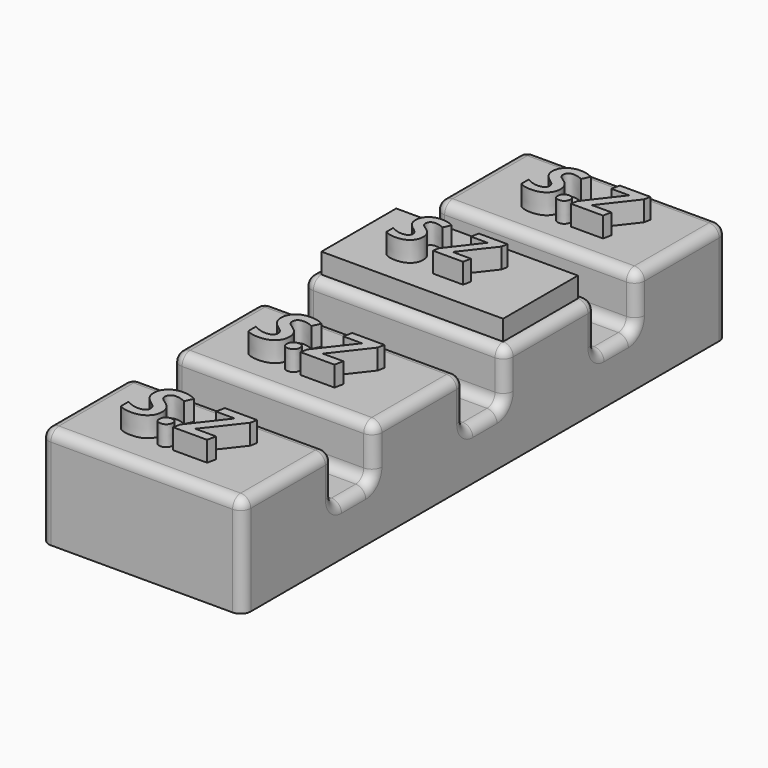
from build123d import *

# Parameters (mm, degrees)
F0_W           = 25.4
F0_H           = 76.2
F1_DEPTH       = 12.7
F2_W           = 6.35
F2_H           = 12.7
F3_DEPTH       = 25.401
F4_F1_R        = 1.27
F4_F2_R        = 1.27
F5_T           = -2.54
F6_TEXT_SIZE   = 7.9179738855
F6_TEXT_SIZE_2 = 8.9047935843
F6_TEXT_SIZE_3 = 8.906235194
F7_DEPTH       = 2.54
F8_TEXT_SIZE   = 8.433056064
F3_FACE_W      = 22.86
F3_FACE_H      = 11.7602
F9_DEPTH       = 2.54


# Not quite as in the source:
# - Text() gives the source's letters only with a copy of the font that has no kerning and outlines rounded to 1/6400 em; it was checked with that copy


with BuildPart() as f1:
    # F0 (on Top) → F1 (new body)
    with BuildSketch(Plane.XY):
        Rectangle(F0_W, F0_H)
    extrude(amount=F1_DEPTH)

    # F2 (on face) → F3 (cut, through all)
    with BuildSketch(Plane.YZ.offset(12.7)):
        with Locations((0, 12.7)):
            Rectangle(F2_W, F2_H)
        with Locations((-20.6502, 12.7)):
            Rectangle(F2_W, F2_H)
        with Locations((20.6502, 12.7)):
            Rectangle(F2_W, F2_H)
    extrude(amount=-F3_DEPTH, mode=Mode.SUBTRACT)

    # F4: fillet of radius 1.27 on 32 edges, made by hand

    # F4_f1
    f4_f1_edges = [f1.edges().sort_by_distance(p)[0] for p in [
        (0, -23.8252, 6.35),
        (0, 3.175, 6.35),
        (0, -3.175, 6.35),
        (0, 23.8252, 6.35),
        (0, 17.4752, 6.35),
        (0, -17.4752, 6.35),
    ]]
    fillet(f4_f1_edges, radius=F4_F1_R)

    # F4_f2
    f4_f2_edges = [f1.edges().sort_by_distance(p)[0] for p in [
        (12.7, -30.9626, 12.7),
        (0, -38.1, 12.7),
        (-12.7, -30.9626, 12.7),
        (0, -23.8252, 12.7),
        (12.7, -10.3251, 12.7),
        (0, -17.4752, 12.7),
        (-12.7, -10.3251, 12.7),
        (0, -3.175, 12.7),
        (12.7, 10.3251, 12.7),
        (0, 3.175, 12.7),
        (-12.7, 10.3251, 12.7),
        (0, 17.4752, 12.7),
        (12.7, 30.9626, 12.7),
        (0, 23.8252, 12.7),
        (-12.7, 30.9626, 12.7),
        (0, 38.1, 12.7),
        (12.7, 0, 6.35),
        (-12.7, 0, 6.35),
        (12.7, 20.6502, 6.35),
        (-12.7, 20.6502, 6.35),
        (12.7, -20.6502, 6.35),
        (-12.7, -20.6502, 6.35),
        (12.7, 38.1, 6.35),
        (12.7, -38.1, 6.35),
        (-12.7, -38.1, 6.35),
        (-12.7, 38.1, 6.35),
        (-12.7, -23.4532256121, 6.7219743879),
        (-12.7, -17.8471743879, 6.7219743879),
        (12.7, -23.4532256121, 6.7219743879),
        (12.7, -17.8471743879, 6.7219743879),
        (-12.7, 17.8471743879, 6.7219743879),
        (-12.7, 23.4532256121, 6.7219743879),
        (12.7, 17.8471743879, 6.7219743879),
        (12.7, 23.4532256121, 6.7219743879),
        (-12.7, -2.8030256121, 6.7219743879),
        (-12.7, 2.8030256121, 6.7219743879),
        (12.7, -2.8030256121, 6.7219743879),
        (12.7, 2.8030256121, 6.7219743879),
    ]]
    fillet(f4_f2_edges, radius=F4_F2_R)

    # F5
    f5_openings = [f1.faces().sort_by_distance(p)[0] for p in [
        (0, 0, 0),
    ]]
    offset(amount=F5_T, openings=f5_openings)

    # F6 (on face) → F7 (join)
    with BuildSketch(Plane.XY.offset(12.7)):
        with Locations((-6.1793054338, 7.6435944065)):
            Text('S.Z', F6_TEXT_SIZE, font='Open Sans', font_style=FontStyle.BOLDITALIC, text_align=(TextAlign.LEFT, TextAlign.BOTTOM))
        with Locations((-6.6630942747, -13.5368104093)):
            Text('S.Z', F6_TEXT_SIZE_2, font='Open Sans', font_style=FontStyle.BOLDITALIC, text_align=(TextAlign.LEFT, TextAlign.BOTTOM))
        with Locations((-6.4476090483, -33.8406581432)):
            Text('S.Z', F6_TEXT_SIZE_3, font='Open Sans', font_style=FontStyle.BOLDITALIC, text_align=(TextAlign.LEFT, TextAlign.BOTTOM))
    extrude(amount=F7_DEPTH)

    # F8 (on face) + F3_face (on face) + F7_face (on face) → F9 (join)
    with BuildSketch(Plane.XY.offset(12.7)):
        with Locations((-5.2801207639, 27.7165938169)):
            Text('S.Z', F8_TEXT_SIZE, font='Open Sans', font_style=FontStyle.BOLDITALIC, text_align=(TextAlign.LEFT, TextAlign.BOTTOM))
    with BuildSketch(Plane(origin=(0, 10.3251, 12.7), x_dir=(1, 0, 0), z_dir=(0, 0, 1))):
        Rectangle(F3_FACE_W, F3_FACE_H)
        with BuildLine():
            add(Edge.make_bspline(
                [(-1.8875161511, -2.2373567458), (-1.8875161511, -2.4959280805), (-1.5707971957, -2.7854290007), (-0.943545202, -2.7854290007), (-0.519191289, -2.3684981883), (-0.519191289, -1.7647526795), (-0.8359102445, -1.4715402091), (-1.4730597056, -1.4715402091), (-1.8875161511, -1.8884710215), (-1.8875161511, -2.2373567458)],
                knots=[0, 0, 0, 1, 2, 3.2139737991, 4.4279475983, 5.3919856152, 6.3560236322, 7.7338704205, 9.1117172089, 9.1117172089, 9.1117172089], degree=2))
        make_face(mode=Mode.SUBTRACT)
        with BuildLine():
            add(Edge.make_bspline(
                [(-6.0209459561, -2.4105624246), (-5.498854553, -2.7594481489), (-3.6665859085, -2.7594481489), (-2.5221912454, -1.81918875), (-2.5221912454, -0.5127230589), (-2.9861350277, 0.2332985432), (-3.4537903604, 0.5425943981)],
                knots=[0, 0, 0, 1, 2.1432706223, 3.2865412446, 3.9921125475, 4.6976838503, 4.6976838503, 4.6976838503], degree=2))
            Line((-6.0209459561, -2.4105624246), (-6.0209459561, -1.3515334174))
            add(Edge.make_bspline(
                [(-4.3965241261, -0.2343567895), (-4.0142344494, -0.5201461594), (-3.821233836, -0.7366532578), (-3.7160732453, -0.987801492), (-3.7160732453, -1.4406106236), (-4.2035235126, -1.7684642298), (-5.274924354, -1.7684642298), (-6.0209459561, -1.3515334174)],
                knots=[0, 0, 0, 1, 2, 3, 4.7111111111, 6.4222222222, 8.9448888889, 8.9448888889, 8.9448888889], degree=2))
            add(Edge.make_bspline(
                [(-1.8875161511, 2.6693126964), (-2.5840504164, 3.051602373), (-3.998151065, 3.051602373), (-4.8839743934, 2.6148766259), (-5.3640015602, 1.8305023379), (-5.3640015602, 0.8989032229), (-4.9309873634, 0.1491700706), (-4.3965241261, -0.2343567895)],
                knots=[0, 0, 0, 1, 1.685840708, 2.3716814159, 3.0575221239, 3.6531654187, 4.2488087134, 4.2488087134, 4.2488087134], degree=2))
            Line((-1.8875161511, 2.6693126964), (-2.3093956972, 1.7686431669))
            add(Edge.make_bspline(
                [(-3.4537903604, 0.5425943981), (-3.897939208, 0.8333325017), (-4.1527989924, 1.1846925928), (-4.1527989924, 1.7067839959), (-3.7432912805, 2.0544325368), (-2.9119040226, 2.0544325368), (-2.3093956972, 1.7686431669)],
                knots=[0, 0, 0, 1, 2, 3.2094240838, 4.4188481675, 6.3473892741, 6.3473892741, 6.3473892741], degree=2))
        make_face(mode=Mode.SUBTRACT)
        Polygon((3.8307456143, -2.6815055935), (0.0375412498, -2.6815055935), (0.1847660767, -1.9045544059), (3.1886474195, 1.9814387151), (1.0891471565, 1.9814387151), (1.2945196041, 2.9711854508), (4.9132811065, 2.9711854508), (4.7549216288, 2.190522713), (1.7312453512, -1.6917588578), (4.036118062, -1.6917588578), align=None, mode=Mode.SUBTRACT)
    with BuildSketch(Plane(origin=(-3.9791969626, 10.4387804644, 15.24), x_dir=(1, 0, 0), z_dir=(0, 0, 1))):
        with BuildLine():
            add(Edge.make_bspline(
                [(-2.0417489934, -2.524242889), (-1.5196575904, -2.8731286133), (0.3126110541, -2.8731286133), (1.4570057172, -1.9328692144), (1.4570057172, -0.6264035233), (0.9930619349, 0.1196180787), (0.5254066022, 0.4289139336)],
                knots=[0, 0, 0, 1, 2.1432706223, 3.2865412446, 3.9921125475, 4.6976838503, 4.6976838503, 4.6976838503], degree=2))
            add(Edge.make_bspline(
                [(0.5254066022, 0.4289139336), (0.0812577546, 0.7196520372), (-0.1736020298, 1.0710121284), (-0.1736020298, 1.5931035315), (0.2359056821, 1.9407520724), (1.06729294, 1.9407520724), (1.6698012654, 1.6549627025)],
                knots=[0, 0, 0, 1, 2, 3.2094240838, 4.4188481675, 6.3473892741, 6.3473892741, 6.3473892741], degree=2))
            Line((1.6698012654, 1.6549627025), (2.0916808115, 2.5556322319))
            add(Edge.make_bspline(
                [(2.0916808115, 2.5556322319), (1.3951465462, 2.9379219086), (-0.0189541024, 2.9379219086), (-0.9047774308, 2.5011961615), (-1.3848045976, 1.7168218734), (-1.3848045976, 0.7852227585), (-0.9517904008, 0.0354896062), (-0.4173271635, -0.3480372539)],
                knots=[0, 0, 0, 1, 1.685840708, 2.3716814159, 3.0575221239, 3.6531654187, 4.2488087134, 4.2488087134, 4.2488087134], degree=2))
            add(Edge.make_bspline(
                [(-0.4173271635, -0.3480372539), (-0.0350374868, -0.6338266238), (0.1579631266, -0.8503337223), (0.2631237173, -1.1014819564), (0.2631237173, -1.554291088), (-0.22432655, -1.8821446942), (-1.2957273914, -1.8821446942), (-2.0417489934, -1.4652138818)],
                knots=[0, 0, 0, 1, 2, 3, 4.7111111111, 6.4222222222, 8.9448888889, 8.9448888889, 8.9448888889], degree=2))
            Line((-2.0417489934, -1.4652138818), (-2.0417489934, -2.524242889))
        make_face()
        Polygon((4.0167382124, -2.7951860579), (7.8099425769, -2.7951860579), (8.0153150246, -1.8054393222), (5.7104423138, -1.8054393222), (8.7341185914, 2.0768422486), (8.8924780691, 2.8575049863), (5.2737165667, 2.8575049863), (5.0683441191, 1.8677582506), (7.1678443821, 1.8677582506), (4.1639630393, -2.0182348704), align=None)
    extrude(amount=F9_DEPTH)


solid = f1.part
